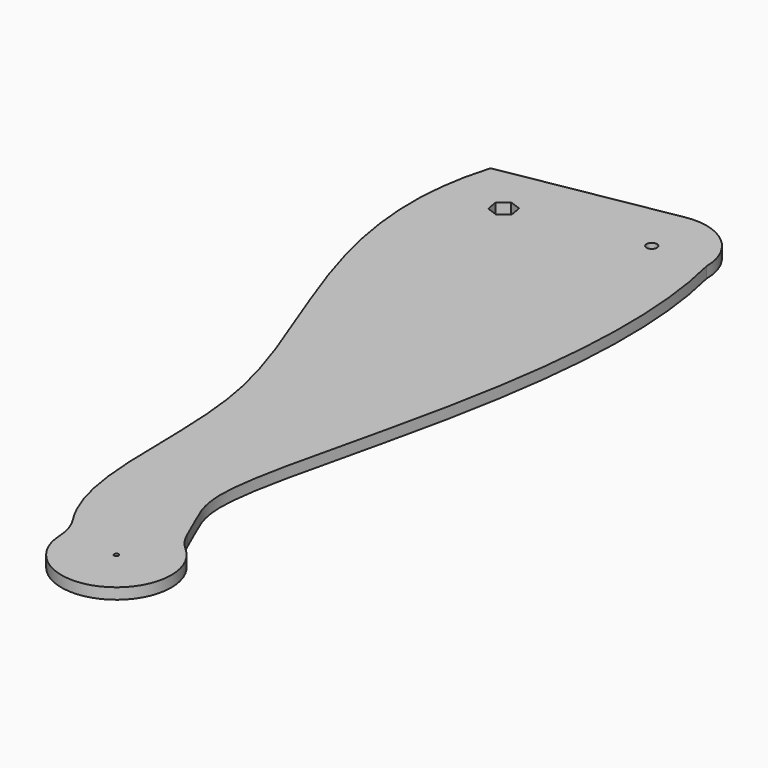
from build123d import *

# Parameters (mm, degrees)
F0_R     = 1
F0_R_2   = 2.35
F2_DEPTH = 5
F3_DEPTH = 5.0010001
F4_R     = 25


with BuildPart() as f2:
    # F0 (on Top) → F2 (new body)
    with BuildSketch(Plane.XY):
        with BuildLine():
            add(Edge.make_bspline(
                [(-82.1230926166, 10.9051483296), (-103.5848878493, -60.0049742057), (-19.3497930189, -169.20375229), (-50.163582636, -268.8476041523), (-24.438918941, -299.5331944222)],
                knots=[0, 0, 0, 0, 0.5562194935, 1, 1, 1, 1], degree=3))
            ThreePointArc((-24.438918941, -299.5331944222), (10.4499069023, -327.5112184995), (11.8990306582, -282.8133433784))
            add(Edge.make_bspline(
                [(25, 0), (47.0782204713, -90.5572716574), (-18.2454262763, -248.1120641616), (7.0555657506, -266.3099283549), (11.8990306582, -282.8133433784)],
                knots=[0, 0, 0, 0, 0.7113740719, 1, 1, 1, 1], degree=3))
            ThreePointArc((25, 0), (16.0696902422, 19.151111078), (-4.3412044417, 24.6201938253))
            Line((-4.3412044417, 24.6201938253), (-82.1230926166, 10.9051483296))
        make_face()
        with Locations((0, -304.8)):
            Circle(F0_R, mode=Mode.SUBTRACT)
        Circle(F0_R_2, mode=Mode.SUBTRACT)
    extrude(amount=F2_DEPTH)

    # F1 (on Top) → F3 (cut, through all)
    with BuildSketch(Plane.XY):
        Polygon((-53.9344131989, -12.2948121673), (-54.886843509, -6.8933114649), (-60.0408954909, -5.0173899577), (-64.2425171626, -8.5429691528), (-63.2900868525, -13.9444698551), (-58.1360348706, -15.8203913624), align=None)
    extrude(amount=F3_DEPTH, mode=Mode.SUBTRACT)

    # F4
    f4_edges = [f2.edges().sort_by_distance(p)[0] for p in [
        (-24.438919, -299.533194, 2.5),
        (11.899031, -282.813343, 2.5),
    ]]
    fillet(f4_edges, radius=F4_R)


solid = f2.part
